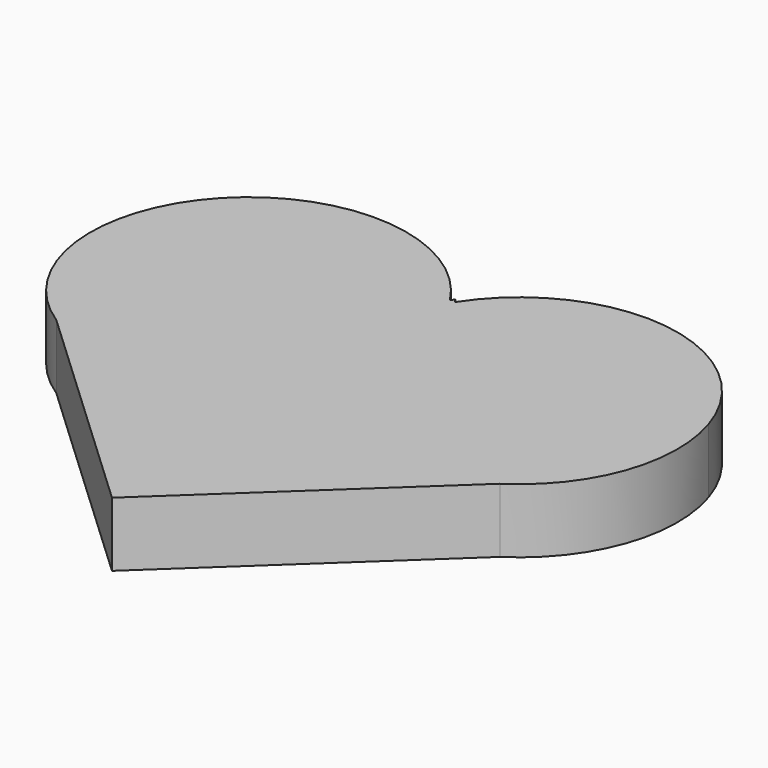
from build123d import *

# Parameters (mm, degrees)
F1_DEPTH = 4.7


# Not quite as in the source:
# - ends of sketch curves that miss each other by under 0.0002 mm in the source are joined


with BuildPart() as f1:
    # F0 (on Top) → F1 (new body)
    with BuildSketch(Plane.XY):
        with BuildLine():
            ThreePointArc((-0.3844762757, 10.7427490547), (-0.4747238326, 10.5966147256), (-0.5627854477, 10.4491528132))
            ThreePointArc((-0.5627854477, 10.4491528132), (-11.7856752997, 15.6525446469), (-21.2647033533, 7.7041756091))
            ThreePointArc((-21.2647033533, 7.7041756091), (-21.1307340877, 0.3344853052), (-16.56156694, -5.4493710653))
            add(Edge.make_bspline(
                [(-16.56156694, -5.4493710653), (-11.1692026058, -10.4978622247), (-5.776839051, -15.5463528768), (-0.3844754963, -20.5948435289)],
                knots=[0, 0, 0, 0, 22.160405753, 22.160405753, 22.160405753, 22.160405753], degree=3))
            add(Edge.make_bspline(
                [(15.7926136092, -5.4493715726), (10.4002500544, -10.4978622247), (5.0078864997, -15.5463528768), (-0.3844754963, -20.5948435289)],
                knots=[0, 0, 0, 0, 22.160405753, 22.160405753, 22.160405753, 22.160405753], degree=3))
            ThreePointArc((15.7926136092, -5.4493715726), (20.3617815363, 0.3344853052), (20.495750802, 7.7041756091))
            ThreePointArc((20.495750802, 7.7041756091), (11.0167227483, 15.6525446469), (-0.2061671036, 10.4491528132))
            ThreePointArc((-0.2061671036, 10.4491528132), (-0.2942287187, 10.5966147256), (-0.3844762757, 10.7427490547))
        make_face()
    extrude(amount=F1_DEPTH)


solid = f1.part
